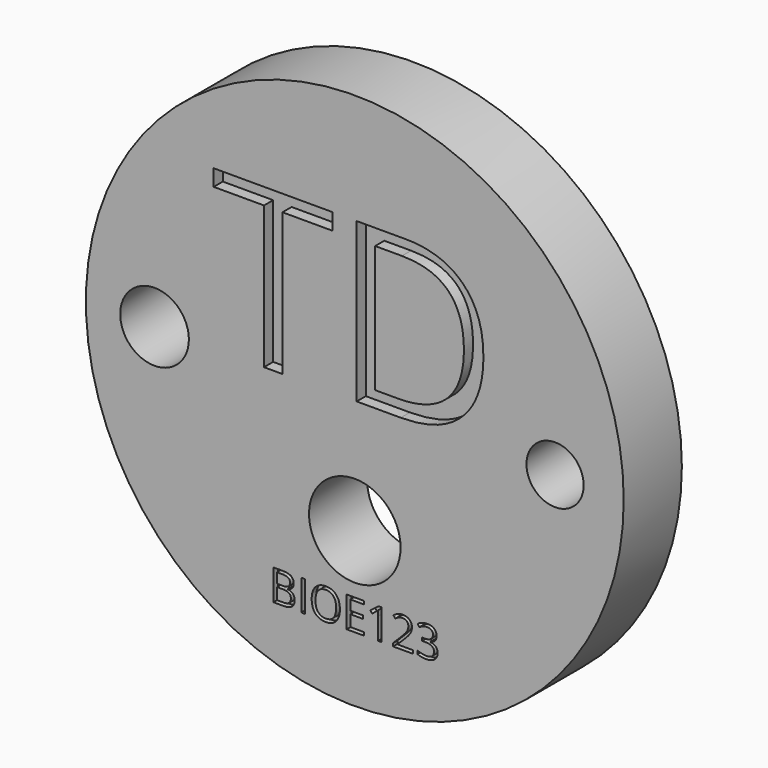
from build123d import *

# Parameters (mm, degrees)
F0_R         = 23.5
F1_DEPTH     = 6.35
F2_R         = 2.5
F2_R_2       = 3
F2_R_3       = 4
F3_DEPTH     = 6.35
F4_TEXT_SIZE = 3.7539013041
F5_DEPTH     = 0.5
F6_TEXT_SIZE = 19.438707326
F7_DEPTH     = 1


# Not quite as in the source:
# - Text() gives the source's letters only with a copy of the font that has no kerning and outlines rounded to 1/6400 em; it was checked with that copy


with BuildPart() as f1:
    # F0 (on Front) → F1 (new body)
    with BuildSketch(Plane.XZ):
        Circle(F0_R)
    extrude(amount=F1_DEPTH)

    # F2 (on face) → F3 (cut)
    with BuildSketch(Plane.XZ.offset(6.35)):
        with Locations((17.5, 0)):
            Circle(F2_R)
        with Locations((-17.5, 0)):
            Circle(F2_R_2)
        with Locations((0, -10)):
            Circle(F2_R_3)
    extrude(amount=-F3_DEPTH, mode=Mode.SUBTRACT)

    # F4 (on face) → F5 (cut)
    with BuildSketch(Plane.XZ.offset(6.35)):
        with Locations((-7.4758357923, -17.8139638156)):
            Text('BIOE123', F4_TEXT_SIZE, font='Open Sans', text_align=(TextAlign.LEFT, TextAlign.BOTTOM))
    extrude(amount=-F5_DEPTH, mode=Mode.SUBTRACT)

    # F6 (on face) → F7 (cut)
    with BuildSketch(Plane.XZ.offset(6.35)):
        with Locations((-12.5, 0)):
            Text('TD', F6_TEXT_SIZE, font='Open Sans', text_align=(TextAlign.LEFT, TextAlign.BOTTOM))
    extrude(amount=-F7_DEPTH, mode=Mode.SUBTRACT)


solid = f1.part
